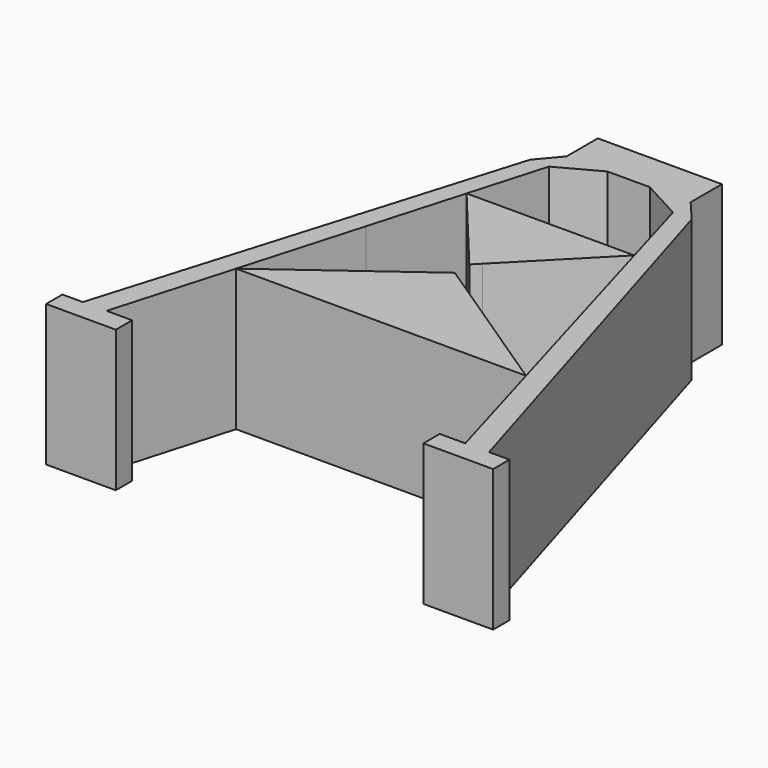
from build123d import *

# Parameters (mm, degrees)
F1_DEPTH = 25.4


with BuildPart() as f1:
    # F0 (on Top) → F1 (new body)
    with BuildSketch(Plane.XY):
        Polygon((-11.1464317888, 47.4868528545), (-14.5056303591, 43.5168929398), (-36.4931114018, -29.4693335891), (-40.1576906443, -29.4693335891), (-40.1576906443, -33.1339128315), (-27.6370421052, -33.1339128315), (-27.6370421052, -29.4693335891), (-32.2177670896, -29.4693335891), (-26.0511616172, -8.1096400765), (-19.8610611523, 13.3314346496), (-15.0670449303, 29.9367968142), (-11.1464317888, 43.5168929398), (-3.8172712084, 47.4868528545), (0, 47.4868528545), (0, 54.5106306672), (-7.4818514986, 54.5106306672), (-11.1464317888, 54.5106306672), align=None)
        Polygon((8.3979964256, 54.5106306672), (0, 54.5106306672), (0, 47.4868528545), (3.8172712084, 47.4868528545), (11.1464317888, 43.5168929398), (15.0670449303, 29.9367968142), (19.8610611523, 13.3314346496), (26.0511616172, -8.1096400765), (32.2177670896, -29.4693335891), (27.6370421052, -29.4693335891), (27.6370421052, -33.1339128315), (40.1576906443, -33.1339128315), (40.1576906443, -29.4693335891), (36.4931114018, -29.4693335891), (14.5056303591, 43.5168929398), (11.1464317888, 47.4868528545), (11.1464317888, 54.5106306672), align=None)
    extrude(amount=F1_DEPTH)


with BuildPart() as f1b:
    # F0 (on Top) → F1, piece 2 (new body)
    with BuildSketch(Plane.XY):
        Polygon((15.0670449303, 29.9367968142), (0, 29.9367968142), (0, 14.6457949804), align=None)
        Polygon((0, 14.6457949804), (0, 29.9367968142), (-15.0670449303, 29.9367968142), (-1.295109789, 13.3314346496), align=None)
    extrude(amount=F1_DEPTH)


with BuildPart() as f1c:
    # F0 (on Top) → F1, piece 3 (new body)
    with BuildSketch(Plane.XY):
        Polygon((0, 9.216254625), (0, -8.1096400765), (26.0511616172, -8.1096400765), align=None)
        Polygon((-1.295109789, 10.0775957108), (-26.0511616172, -8.1096400765), (0, -8.1096400765), (0, 9.216254625), align=None)
    extrude(amount=F1_DEPTH)


solid = Compound([f1.part, f1b.part, f1c.part])
